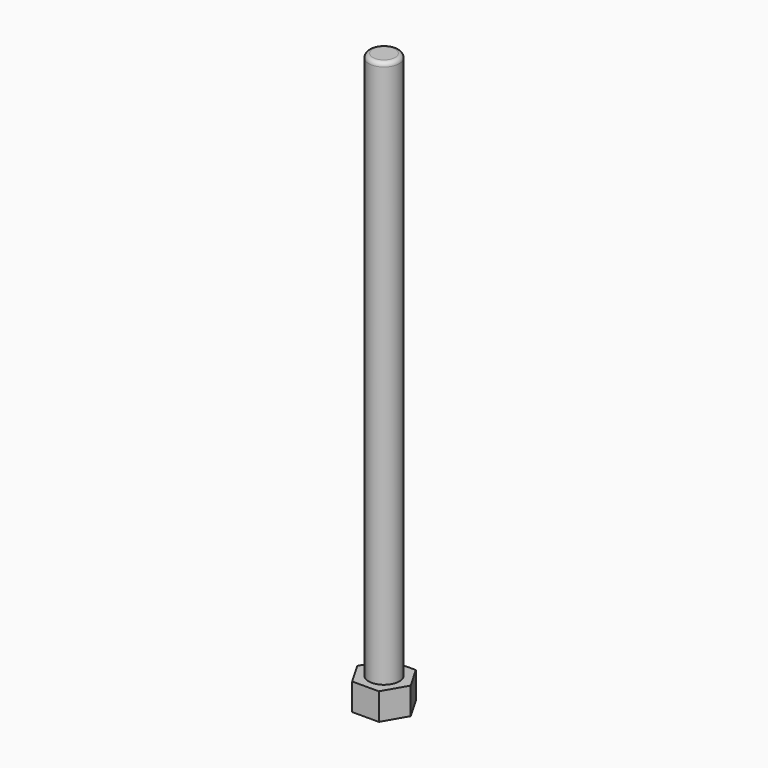
from build123d import *

# Parameters (mm, degrees)
F0_R     = 4.74599
F1_DEPTH = 177.8
F3_DEPTH = 8.334375
F4_R     = 1.27


# Not quite as in the source:
# - a length typed as a fraction of an inch, garbled in the dataset ("3 / 203.2 mm" for 3/8 in), is restored


with BuildPart() as f1:
    # F0 (on Top) → F1 (new body)
    with BuildSketch(Plane.XY):
        Circle(F0_R)
    extrude(amount=F1_DEPTH)

    # F2 (on Top) → F3 (join)
    with BuildSketch(Plane.XY):
        Polygon((-4.1244459855, -7.14375), (4.1244459855, -7.14375), (8.248891971, 0), (4.1244459855, 7.14375), (-4.1244459855, 7.14375), (-8.248891971, 0), align=None)
    extrude(amount=F3_DEPTH)

    # F4
    f4_edges = [f1.edges().sort_by_distance(p)[0] for p in [
        (-4.74599, 0, 177.8),
    ]]
    fillet(f4_edges, radius=F4_R)


solid = f1.part
